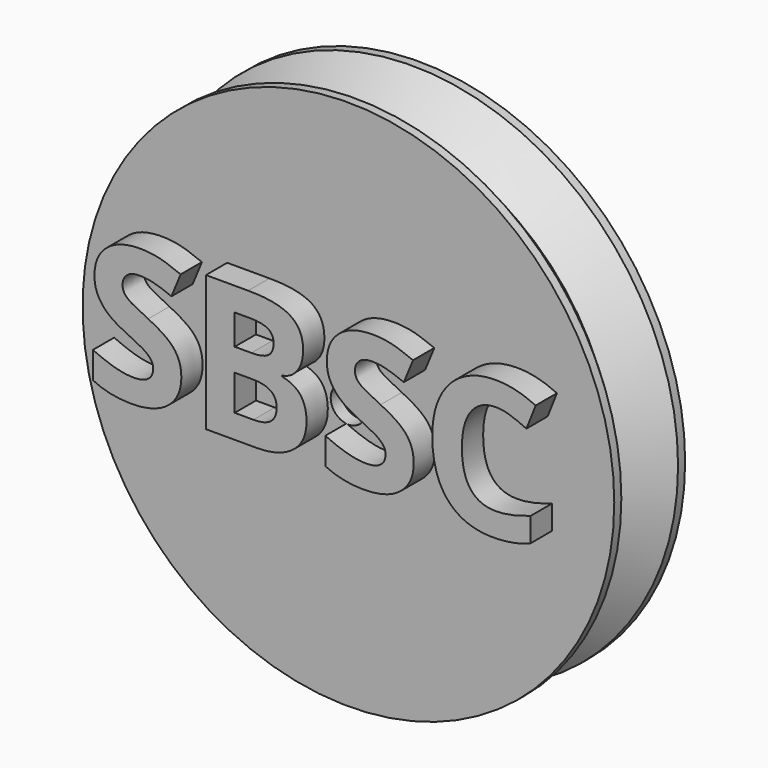
from build123d import *

# Parameters (mm, degrees)
F0_R         = 15
F1_DEPTH     = 2.5
F2_SIZE      = 2
F3_R         = 15
F3_R_2       = 13
F4_DEPTH     = 2.5
F5_SIZE      = 1.99999
F6_R         = 1
F7_DEPTH     = 0.75
F8_TEXT_SIZE = 10.7248842445
F9_DEPTH     = 1.5


# Not quite as in the source:
# - a fillet or chamfer is up to 0.001 mm smaller than in the source, because OpenCascade refuses the exact size
# - Text() gives the source's letters only with a copy of the font that has no kerning and outlines rounded to 1/6400 em; it was checked with that copy


with BuildPart() as f1:
    # F0 (on Front) → F1 (new body)
    with BuildSketch(Plane.XZ):
        Circle(F0_R)
    extrude(amount=F1_DEPTH)

    # F2
    f2_edges = [f1.edges().sort_by_distance(p)[0] for p in [
        (-15, -2.5, 0),
    ]]
    chamfer(f2_edges, length=F2_SIZE)

    # F3 (on face) → F4 (join)
    with BuildSketch(Plane.XZ.offset(2.5)):
        Circle(F3_R)
        Circle(F3_R_2, mode=Mode.SUBTRACT)
        Circle(F3_R_2)
    extrude(amount=F4_DEPTH)

    # F5 (size 2 in the source; OpenCascade refuses exactly that, so slightly less here)
    f5_edges = [f1.edges().sort_by_distance(p)[0] for p in [
        (-15, -2.5, 0),
    ]]
    chamfer(f5_edges, length=F5_SIZE)

    # F6 (on face) → F7 (cut)
    with BuildSketch(Plane.XZ.offset(5)):
        Circle(F6_R)
    extrude(amount=-F7_DEPTH, mode=Mode.SUBTRACT)

    # F8 (on face) → F9 (join)
    with BuildSketch(Plane.XZ.offset(5)):
        with Locations((-13.7116839178, -2.8447520453)):
            Text('SBSC', F8_TEXT_SIZE, font='Open Sans', font_style=FontStyle.BOLD, text_align=(TextAlign.LEFT, TextAlign.BOTTOM))
    extrude(amount=F9_DEPTH)


solid = f1.part
